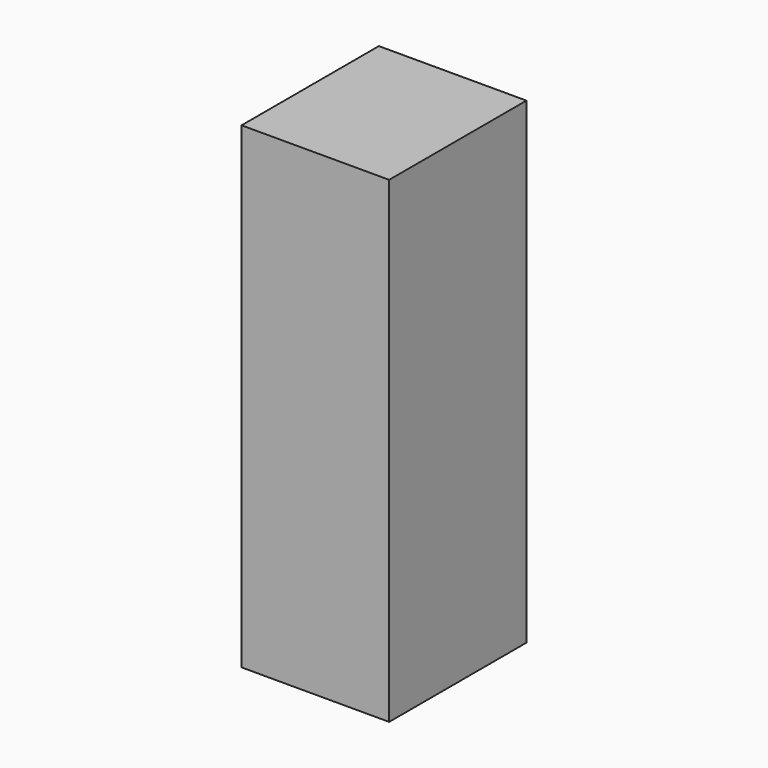
from build123d import *

# Parameters (mm, degrees)
F0_W     = 21.8467004597
F0_H     = 70.6471279263
F1_DEPTH = 25.4


# Not quite as in the source:
# - a feature of the source that left no trace in its solid (it failed there, or was rolled back) is left out


with BuildPart() as f1:
    # F0 (on Front) → F1 (new body)
    with BuildSketch(Plane.XZ):
        with Locations((-37.8770735115, 3.8302652538)):
            Rectangle(F0_W, F0_H)
    extrude(amount=F1_DEPTH)


solid = f1.part
